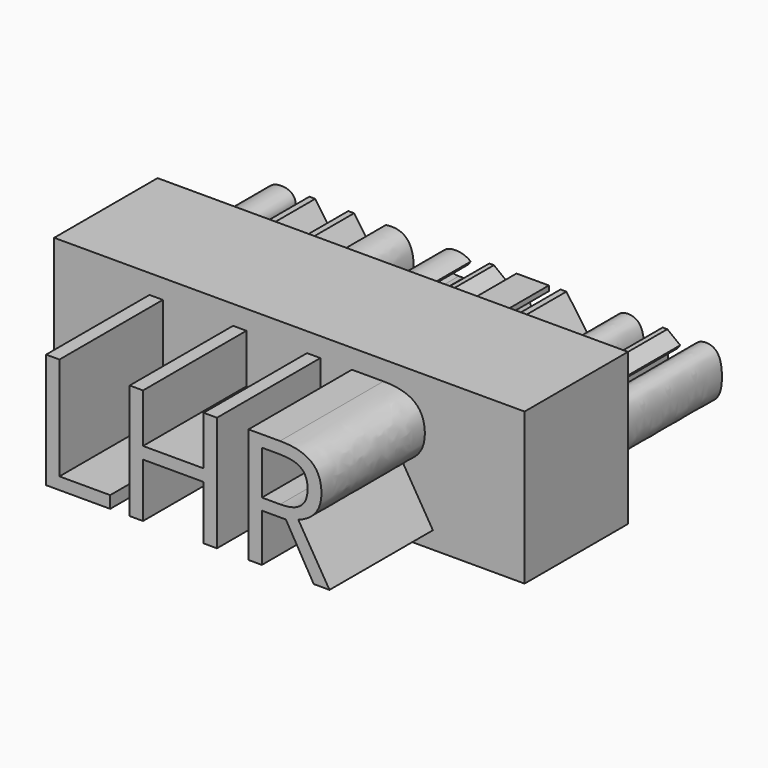
from build123d import *

# Parameters (mm, degrees)
F0_W         = 92.453956604
F0_H         = 29.7733061016
F1_DEPTH     = 25.4
F2_TEXT_SIZE = 31.6532574491
F3_DEPTH     = 25.4
F5_TEXT_SIZE = 13.3796781277
F6_DEPTH     = 25.4


# Not quite as in the source:
# - Text() gives the source's letters only with a copy of the font that has no kerning and outlines rounded to 1/6400 em; it was checked with that copy


with BuildPart() as f1:
    # F0 (on Front) → F1 (new body)
    with BuildSketch(Plane.XZ):
        with Locations((46.226978302, 14.8866530508)):
            Rectangle(F0_W, F0_H)
    extrude(amount=F1_DEPTH)

    # F2 (on face) → F3 (join)
    with BuildSketch(Plane.XZ.offset(25.4)):
        with Locations((15.6236386392, 3.3780355006)):
            Text('LHR', F2_TEXT_SIZE, font='Open Sans', text_align=(TextAlign.LEFT, TextAlign.BOTTOM))
    extrude(amount=F3_DEPTH)

    # F5 (on face) → F6 (join)
    with BuildSketch(Plane(origin=(0, 0, 0), x_dir=(-1, 0, 0), z_dir=(0, 1, 0))):
        with Locations((-91.2724011526, 9.7238911333)):
            Text('010 4713 6448', F5_TEXT_SIZE, font='Open Sans', text_align=(TextAlign.LEFT, TextAlign.BOTTOM))
    extrude(amount=F6_DEPTH)


solid = f1.part
